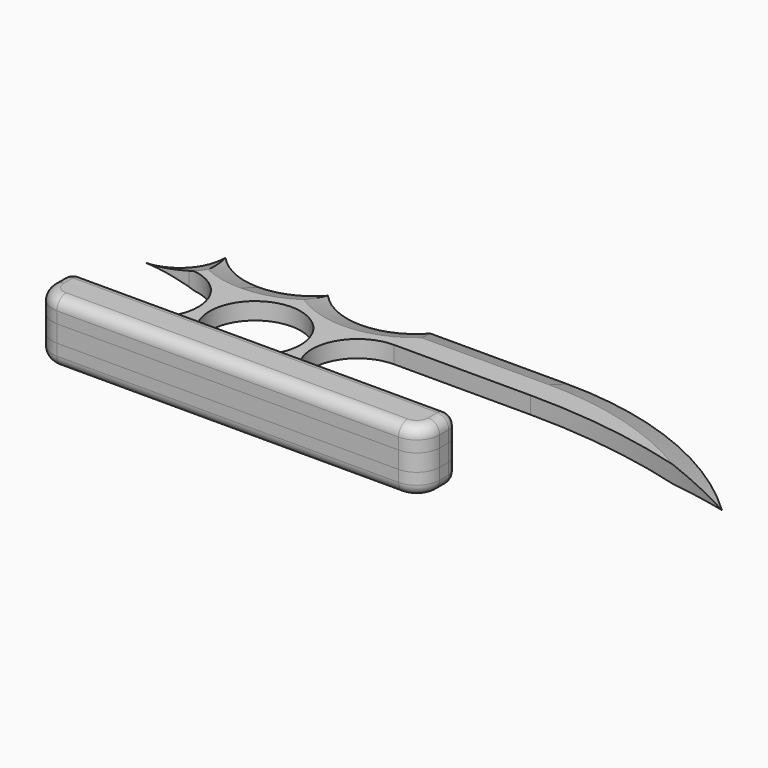
from build123d import *

# Parameters (mm, degrees)
F0_R     = 12.7
F1_DEPTH = 4.7625
F3_START = 4.7625
F3_DEPTH = 6.35
F4_DEPTH = 6.35
F5_R     = 3.175
F5_2_R   = 3.175
F6_SIZE2 = 6.35
F6_SIZE  = 2.38125
F7_SIZE2 = 2.38124
F7_SIZE  = 6.34999


# Not quite as in the source:
# - a fillet or chamfer is up to 0.001 mm smaller than in the source, because OpenCascade refuses the exact size


with BuildPart() as f1:
    # F0 (on Top) → F1 (new body)
    with BuildSketch(Plane.XY):
        with BuildLine():
            Line((63.5, 0), (28.575, 0))
            ThreePointArc((28.575, 0), (15.875, 12.7), (28.575, 25.4))
            Line((28.575, 25.4), (66.675, 25.4))
            ThreePointArc((66.675, 25.4), (99.0537739113, 22.1938695566), (130.175, 12.7))
            ThreePointArc((130.175, 12.7), (100.8707965253, 31.5144913133), (66.675, 38.1))
            Line((66.675, 38.1), (28.575, 38.1))
            ThreePointArc((28.575, 38.1), (14.2875, 31.75), (0, 38.1))
            ThreePointArc((0, 38.1), (-6.4699695128, 33.408993013), (-14.2875007235, 31.75))
            ThreePointArc((-14.2875007235, 31.75), (-22.1050316037, 33.4089930196), (-28.5750007235, 38.1))
            ThreePointArc((-28.5750007235, 38.1), (-32.2947446025, 29.1197438789), (-41.2750007235, 25.4))
            Line((-41.2750007235, 25.4), (-28.5750007235, 25.4))
            ThreePointArc((-28.5750007235, 25.4), (-15.8750007235, 12.7), (-28.5750007235, 0))
            Line((-28.5750007235, 0), (-38.1000007235, 0))
            ThreePointArc((-38.1000007235, 0), (-40.3450647538, -0.9299359697), (-41.2750007235, -3.175))
            Line((-41.2750007235, -3.175), (-41.2750007235, -6.35))
            ThreePointArc((-41.2750007235, -6.35), (-39.4151287841, -10.8401280605), (-34.9250007235, -12.7))
            Line((-34.9250007235, -12.7), (60.325, -12.7))
            ThreePointArc((60.325, -12.7), (64.8151280605, -10.8401280605), (66.675, -6.35))
            Line((66.675, -6.35), (66.675, -3.175))
            ThreePointArc((66.675, -3.175), (65.7450640303, -0.9299359697), (63.5, 0))
        make_face()
        with Locations((0, 12.7)):
            Circle(F0_R, mode=Mode.SUBTRACT)
    extrude(amount=F1_DEPTH)

    # F6
    f6_edges = [f1.edges().sort_by_distance(p)[0] for p in [
        (47.625, 38.1, 4.7625),
        (14.2875, 31.75, 4.7625),
        (100.870797, 31.514491, 4.7625),
        (-22.105032, 33.408993, 4.7625),
        (-6.46997, 33.408993, 4.7625),
        (-32.294745, 29.119744, 4.7625),
    ]]
    chamfer(f6_edges, length=F6_SIZE, length2=F6_SIZE2)

    # F7 (size 6.35 and 2.38125 in the source; OpenCascade refuses exactly that, so slightly less here)
    f7_edges = [f1.edges().sort_by_distance(p)[0] for p in [
        (-32.294745, 29.119744, 0),
        (-22.105032, 33.408993, 0),
        (-6.46997, 33.408993, 0),
        (14.2875, 31.75, 0),
        (47.625, 38.1, 0),
        (100.870797, 31.514491, 0),
    ]]
    f7_side = f1.faces().sort_by_distance((-31.030313, 27.855312, 0))[0]
    chamfer(f7_edges, length=F7_SIZE, length2=F7_SIZE2, reference=f7_side)


with BuildPart() as f3:
    # F2 (on Top) → F3 (new body)
    with BuildSketch(Plane.XY.offset(F3_START)):
        with BuildLine():
            Line((63.5, 0), (-38.1, 0))
            ThreePointArc((-38.1, 0), (-40.3450640303, -0.9299359697), (-41.275, -3.175))
            Line((-41.275, -3.175), (-41.275, -6.35))
            ThreePointArc((-41.275, -6.35), (-39.4151280605, -10.8401280605), (-34.925, -12.7))
            Line((-34.925, -12.7), (60.325, -12.7))
            ThreePointArc((60.325, -12.7), (64.8151280605, -10.8401280605), (66.675, -6.35))
            Line((66.675, -6.35), (66.675, -3.175))
            ThreePointArc((66.675, -3.175), (65.7450640303, -0.9299359697), (63.5, 0))
        make_face()
    extrude(amount=F3_DEPTH)

    # F5
    f5_edges = [f3.edges().sort_by_distance(p)[0] for p in [
        (12.7, 0, 11.1125),
        (-40.345064, -0.929936, 11.1125),
        (-41.275, -4.7625, 11.1125),
        (-39.415128, -10.840128, 11.1125),
        (12.7, -12.7, 11.1125),
        (64.815128, -10.840128, 11.1125),
        (66.675, -4.7625, 11.1125),
        (65.745064, -0.929936, 11.1125),
    ]]
    fillet(f5_edges, radius=F5_R)


with BuildPart() as f4:
    # F2 (on Top) → F4 (new body)
    with BuildSketch(Plane.XY):
        with BuildLine():
            Line((63.5, 0), (-38.1, 0))
            ThreePointArc((-38.1, 0), (-40.3450640303, -0.9299359697), (-41.275, -3.175))
            Line((-41.275, -3.175), (-41.275, -6.35))
            ThreePointArc((-41.275, -6.35), (-39.4151280605, -10.8401280605), (-34.925, -12.7))
            Line((-34.925, -12.7), (60.325, -12.7))
            ThreePointArc((60.325, -12.7), (64.8151280605, -10.8401280605), (66.675, -6.35))
            Line((66.675, -6.35), (66.675, -3.175))
            ThreePointArc((66.675, -3.175), (65.7450640303, -0.9299359697), (63.5, 0))
        make_face()
    extrude(amount=-F4_DEPTH)

    # F5#2
    f5_2_edges = [f4.edges().sort_by_distance(p)[0] for p in [
        (12.7, 0, -6.35),
        (-40.345064, -0.929936, -6.35),
        (-41.275, -4.7625, -6.35),
        (-39.415128, -10.840128, -6.35),
        (12.7, -12.7, -6.35),
        (64.815128, -10.840128, -6.35),
        (66.675, -4.7625, -6.35),
        (65.745064, -0.929936, -6.35),
    ]]
    fillet(f5_2_edges, radius=F5_2_R)


solid = Compound([f1.part, f3.part, f4.part])
